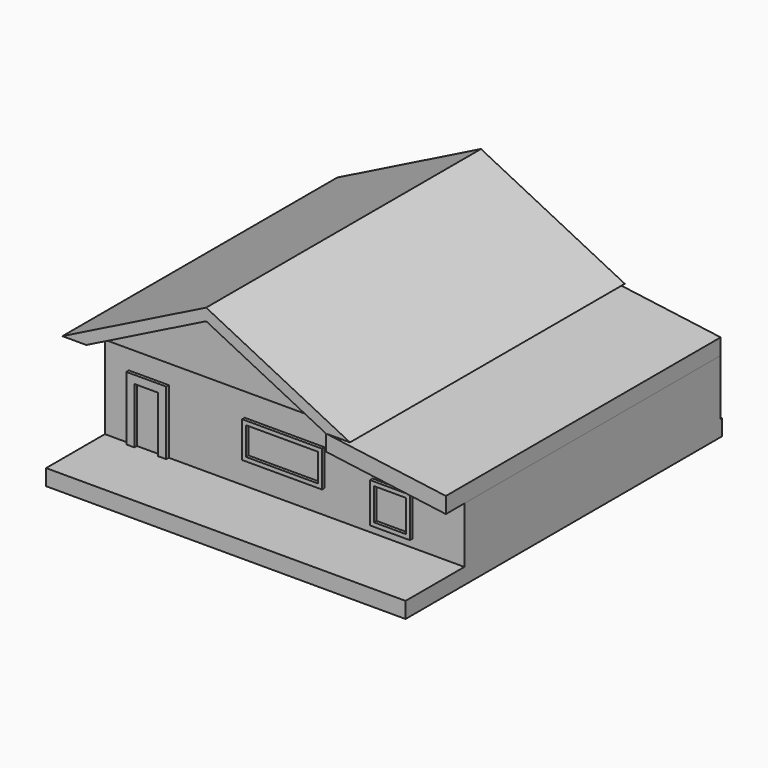
from build123d import *

# Parameters (mm, degrees)
F1_DEPTH      = 914.4
F1_DEPTH_BACK = 12192
F2_DEPTH      = 304.8
F2_DEPTH_BACK = 12192
F0_W          = 3048
F0_H          = 1371.6
F0_W_2        = 1524
F0_H_2        = 1524
F0_W_3        = 2743.2
F0_H_3        = 1066.8
F0_W_4        = 1219.2
F0_H_4        = 1219.2
F0_W_5        = 914.4
F0_H_5        = 2133.6
F3_DEPTH      = 30.48
F3_DEPTH_BACK = 12192
F4_DEPTH      = 152.4
F0_W_6        = 4572
F0_H_6        = 609.6
F5_DEPTH      = 2834.64
F5_DEPTH_BACK = 12252.96


# Not quite as in the source:
# - the program builds the solid bodies; features that only make, move or delete a surface that nothing else refers to are left out


with BuildPart() as f1:
    # F0 (on Front) → F1 (new body, two sides)
    with BuildSketch(Plane.XZ) as f1_sk:
        Polygon((-5486.4, 1676.4), (-4572, 1676.4), (0, 3962.4), (0, 4419.6), align=None)
        Polygon((0, 4419.6), (0, 3962.4), (4572, 1676.4), (5486.4, 1676.4), align=None)
    extrude(amount=F1_DEPTH)
    extrude(f1_sk.sketch, amount=-F1_DEPTH_BACK)



with BuildPart() as f1b:
    # F0 (on Front) → F1, piece 2 (new body, two sides)
    with BuildSketch(Plane.XZ) as f1_2_sk:
        Polygon((9144, 1066.8), (4572, 1676.4), (4572, 1066.8), (9144, 457.2), align=None)
    extrude(amount=F1_DEPTH)
    extrude(f1_2_sk.sketch, amount=-F1_DEPTH_BACK)


with BuildPart() as f1_1:
    add(f1.part)

    add(f1b.part)  # F2 merges F1b
    # F0 (on Front) → F2 (join, two sides)
    with BuildSketch(Plane.XZ) as f2_sk:
        Polygon((0, 3962.4), (-4572, 1676.4), (0, 1676.4), align=None)
        Polygon((0, 3962.4), (0, 1676.4), (4572, 1676.4), align=None)
    extrude(amount=F2_DEPTH)
    extrude(f2_sk.sketch, amount=-F2_DEPTH_BACK)


with BuildPart() as f3:
    # F0 (on Front) → F3 (new body, two sides)
    with BuildSketch(Plane.XZ) as f3_sk:
        Polygon((0, 1676.4), (-4572, 1676.4), (-4572, -1676.4), (-3657.6, -1676.4), (-3657.6, 762), (-2133.6, 762), (-2133.6, -1676.4), (4572, -1676.4), (4572, 1066.8), (4572, 1676.4), align=None)
        with Locations((2286, -76.2)):
            Rectangle(F0_W, F0_H, mode=Mode.SUBTRACT)
        Polygon((9144, 457.2), (4572, 1066.8), (4572, -1676.4), (9144, -1676.4), align=None)
        with Locations((6400.8, -609.6)):
            Rectangle(F0_W_2, F0_H_2, mode=Mode.SUBTRACT)
        with Locations((2286, -76.2)):
            Rectangle(F0_W, F0_H)
        with Locations((2286, -76.2)):
            Rectangle(F0_W_3, F0_H_3, mode=Mode.SUBTRACT)
        with Locations((2286, -76.2)):
            Rectangle(F0_W_3, F0_H_3)
        with Locations((6400.8, -609.6)):
            Rectangle(F0_W_2, F0_H_2)
        with Locations((6400.8, -609.6)):
            Rectangle(F0_W_4, F0_H_4, mode=Mode.SUBTRACT)
        with Locations((-2895.6, -609.6)):
            Rectangle(F0_W_5, F0_H_5)
        Polygon((-3657.6, 762), (-3657.6, -1676.4), (-3352.8, -1676.4), (-3352.8, 457.2), (-2438.4, 457.2), (-2438.4, -1676.4), (-2133.6, -1676.4), (-2133.6, 762), align=None)
        with Locations((6400.8, -609.6)):
            Rectangle(F0_W_4, F0_H_4)
    extrude(amount=F3_DEPTH)
    extrude(f3_sk.sketch, amount=-F3_DEPTH_BACK)

    # F0 (on Front) → F4 (join)
    with BuildSketch(Plane.XZ):
        Polygon((-3657.6, 762), (-3657.6, -1676.4), (-3352.8, -1676.4), (-3352.8, 457.2), (-2438.4, 457.2), (-2438.4, -1676.4), (-2133.6, -1676.4), (-2133.6, 762), align=None)
        with Locations((2286, -76.2)):
            Rectangle(F0_W, F0_H)
        with Locations((2286, -76.2)):
            Rectangle(F0_W_3, F0_H_3, mode=Mode.SUBTRACT)
        with Locations((6400.8, -609.6)):
            Rectangle(F0_W_2, F0_H_2)
        with Locations((6400.8, -609.6)):
            Rectangle(F0_W_4, F0_H_4, mode=Mode.SUBTRACT)
    extrude(amount=F4_DEPTH)

    # F0 (on Front) → F5 (join, two sides)
    with BuildSketch(Plane.XZ) as f5_sk:
        with Locations((6858, -1981.2)):
            Rectangle(F0_W_6, F0_H_6)
        Polygon((-3657.6, -1676.4), (-4572, -1676.4), (-4572, -2286), (4572, -2286), (4572, -1676.4), (-2133.6, -1676.4), (-2438.4, -1676.4), (-3352.8, -1676.4), align=None)
    extrude(amount=F5_DEPTH)
    extrude(f5_sk.sketch, amount=-F5_DEPTH_BACK)


solid = Compound([f1_1.part, f3.part])
